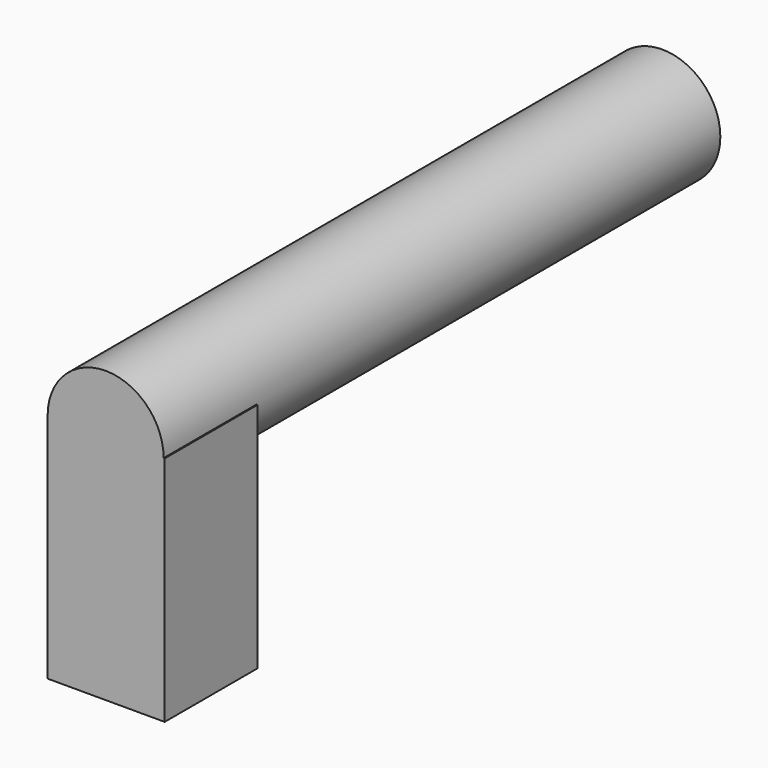
from build123d import *

# Parameters (mm, degrees)
F1_R     = 12.7
F2_DEPTH = 152.4
F4_DEPTH = 25.4


with BuildPart() as f2:
    # F1 (on face) → F2 (new body)
    with BuildSketch(Plane.XZ):
        with Locations((-27.7367867529, 61.1216872931)):
            Circle(F1_R)
    extrude(amount=F2_DEPTH)

    # F3 (on face) → F4 (join)
    with BuildSketch(Plane.XZ.offset(152.4)):
        with BuildLine():
            Line((-14.8034961894, 61.1216872931), (-15.0367867529, 61.1216872931))
            ThreePointArc((-15.0367867529, 61.1216872931), (-27.7367867529, 48.4216872931), (-40.4367867529, 61.1216872931))
            Line((-40.4367867529, 61.1216872931), (-40.4367867529, 10.3216872931))
            Line((-40.4367867529, 10.3216872931), (-14.8034961894, 10.3216872931))
            Line((-14.8034961894, 10.3216872931), (-14.8034961894, 61.1216872931))
        make_face()
    extrude(amount=-F4_DEPTH)


solid = f2.part
